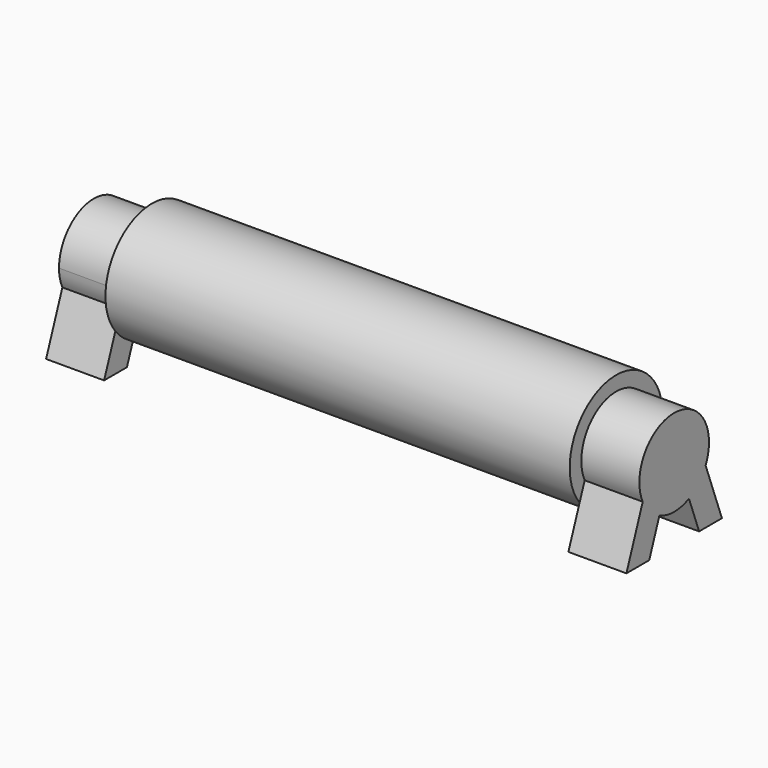
from build123d import *

# Parameters (mm, degrees)
F0_R          = 250
F1_DEPTH      = 2000
F2_R          = 125
F3_DEPTH      = 250
F3_DEPTH_BACK = 2250
F4_R          = 125
F5_DEPTH      = 250
F6_R          = 125
F7_DEPTH      = 250


with BuildPart() as f1:
    # F0 (on Right) → F1 (new body)
    with BuildSketch(Plane.YZ):
        Circle(F0_R)
    extrude(amount=F1_DEPTH)

    # F2 (on face) → F3 (join, two sides)
    with BuildSketch(Plane.YZ.offset(2000)) as f3_sk:
        Circle(F2_R)
    extrude(amount=F3_DEPTH)
    extrude(f3_sk.sketch, amount=-F3_DEPTH_BACK)

    # F4 (on face) → F5 (join)
    with BuildSketch(Plane.YZ.offset(2000)):
        with BuildLine():
            ThreePointArc((169.3175568296, -80.5469735573), (182.897911286, -41.2868507787), (187.5, 0))
            ThreePointArc((187.5, 0), (-41.2868507787, 182.897911286), (-169.3175568296, -80.5469735573))
            ThreePointArc((-169.3175568296, -80.5469735573), (-132.229157972, -132.9349456765), (-79.6444930507, -169.7439387039))
            ThreePointArc((-79.6444930507, -169.7439387039), (0, -187.5), (79.6444930507, -169.7439387039))
            ThreePointArc((79.6444930507, -169.7439387039), (132.229157972, -132.9349456765), (169.3175568296, -80.5469735573))
        make_face()
        Circle(F4_R, mode=Mode.SUBTRACT)
        with BuildLine():
            ThreePointArc((-79.6444930507, -169.7439387039), (-132.229157972, -132.9349456765), (-169.3175568296, -80.5469735573))
            Line((-169.3175568296, -80.5469735573), (-196.7506873322, -154.2373723658))
            ThreePointArc((-196.7506873322, -154.2373723658), (-153.6770038013, -197.1886875626), (-101.505253912, -228.4659349405))
            Line((-101.505253912, -228.4659349405), (-79.6444930507, -169.7439387039))
        make_face()
        with BuildLine():
            Line((196.7506873322, -154.2373723658), (169.3175568296, -80.5469735573))
            ThreePointArc((169.3175568296, -80.5469735573), (132.229157972, -132.9349456765), (79.6444930507, -169.7439387039))
            Line((79.6444930507, -169.7439387039), (101.505253912, -228.4659349405))
            ThreePointArc((101.505253912, -228.4659349405), (153.6770038013, -197.1886875626), (196.7506873322, -154.2373723658))
        make_face()
        with BuildLine():
            ThreePointArc((-101.505253912, -228.4659349405), (-153.6770038013, -197.1886875626), (-196.7506873322, -154.2373723658))
            Line((-196.7506873322, -154.2373723658), (-257.1270477757, -316.4193034172))
            Line((-257.1270477757, -316.4193034172), (-134.2481386646, -316.4193034172))
            Line((-134.2481386646, -316.4193034172), (-101.505253912, -228.4659349405))
        make_face()
        with BuildLine():
            Line((257.1270477757, -316.4193034172), (196.7506873322, -154.2373723658))
            ThreePointArc((196.7506873322, -154.2373723658), (153.6770038013, -197.1886875626), (101.505253912, -228.4659349405))
            Line((101.505253912, -228.4659349405), (134.2481386646, -316.4193034172))
            Line((134.2481386646, -316.4193034172), (257.1270477757, -316.4193034172))
        make_face()
    extrude(amount=F5_DEPTH)

    # F6 (on face) → F7 (join)
    with BuildSketch(Plane(origin=(0, 0, 0), x_dir=(0, -1, 0), z_dir=(-1, 0, 0))):
        with BuildLine():
            ThreePointArc((-101.505253912, -228.4659349405), (-153.6770038013, -197.1886875626), (-196.7506873322, -154.2373723658))
            Line((-196.7506873322, -154.2373723658), (-257.1270477757, -316.4193034172))
            Line((-257.1270477757, -316.4193034172), (-134.2481386646, -316.4193034172))
            Line((-134.2481386646, -316.4193034172), (-101.505253912, -228.4659349405))
        make_face()
        with BuildLine():
            Line((257.1270477757, -316.4193034172), (196.7506873322, -154.2373723658))
            ThreePointArc((196.7506873322, -154.2373723658), (153.6770038013, -197.1886875626), (101.505253912, -228.4659349405))
            Line((101.505253912, -228.4659349405), (134.2481386646, -316.4193034172))
            Line((134.2481386646, -316.4193034172), (257.1270477757, -316.4193034172))
        make_face()
        with BuildLine():
            Line((196.7506873322, -154.2373723658), (169.3175568296, -80.5469735573))
            ThreePointArc((169.3175568296, -80.5469735573), (132.229157972, -132.9349456765), (79.6444930507, -169.7439387039))
            Line((79.6444930507, -169.7439387039), (101.505253912, -228.4659349405))
            ThreePointArc((101.505253912, -228.4659349405), (153.6770038013, -197.1886875626), (196.7506873322, -154.2373723658))
        make_face()
        with BuildLine():
            ThreePointArc((-79.6444930507, -169.7439387039), (-132.229157972, -132.9349456765), (-169.3175568296, -80.5469735573))
            Line((-169.3175568296, -80.5469735573), (-196.7506873322, -154.2373723658))
            ThreePointArc((-196.7506873322, -154.2373723658), (-153.6770038013, -197.1886875626), (-101.505253912, -228.4659349405))
            Line((-101.505253912, -228.4659349405), (-79.6444930507, -169.7439387039))
        make_face()
        with BuildLine():
            ThreePointArc((187.5, 0), (-41.2868507787, 182.897911286), (-169.3175568296, -80.5469735573))
            ThreePointArc((-169.3175568296, -80.5469735573), (-132.229157972, -132.9349456765), (-79.6444930507, -169.7439387039))
            ThreePointArc((-79.6444930507, -169.7439387039), (0, -187.5), (79.6444930507, -169.7439387039))
            ThreePointArc((79.6444930507, -169.7439387039), (132.229157972, -132.9349456765), (169.3175568296, -80.5469735573))
            ThreePointArc((169.3175568296, -80.5469735573), (182.897911286, -41.2868507787), (187.5, 0))
        make_face()
        Circle(F6_R, mode=Mode.SUBTRACT)
    extrude(amount=F7_DEPTH)


solid = f1.part
